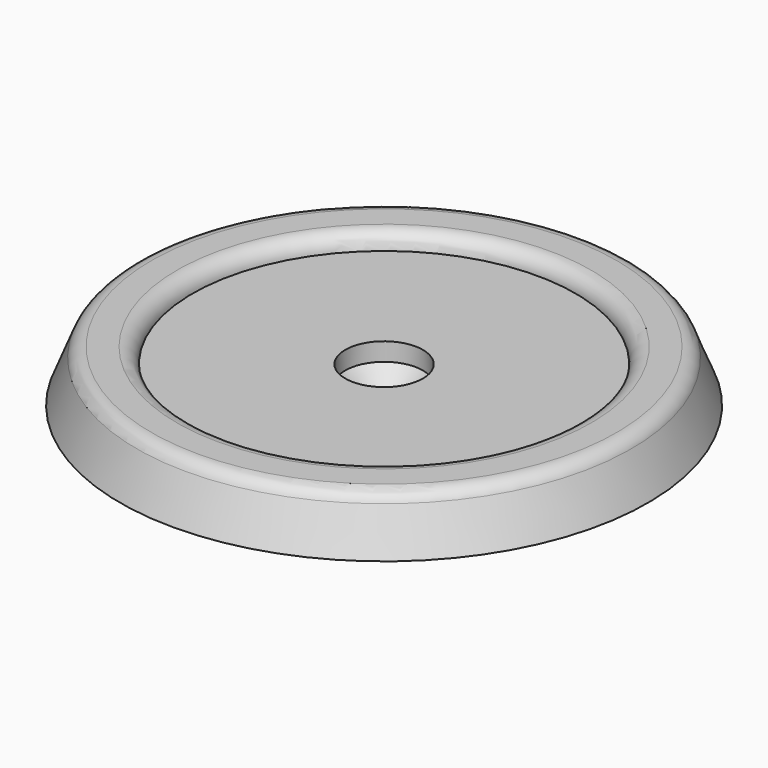
from build123d import *

# Parameters (mm, degrees)
F0_R        = 18.5
F0_R_2      = 2
F1_DEPTH    = 3.5
F2_R        = 3.75
F3_DEPTH    = 0.5
F4_S5_R     = 3.75
F4_T6_DEPTH = 9
F8_R        = 1.49999


# Not quite as in the source:
# - a fillet or chamfer that OpenCascade refuses, or shapes differently, is made with other operations: its cross-section is extruded or revolved along the edge and cut away or added
# - a fillet or chamfer is up to 0.001 mm smaller than in the source, because OpenCascade refuses the exact size


with BuildPart() as f1:
    # F0 (on Top) → F1 (new body)
    with BuildSketch(Plane.XY):
        Circle(F0_R)
        Circle(F0_R_2, mode=Mode.SUBTRACT)
    extrude(amount=F1_DEPTH)

    # F2 (on face) → F3 (cut)
    with BuildSketch(Plane.XY.offset(3.5)):
        Circle(F2_R)
    extrude(amount=-F3_DEPTH, mode=Mode.SUBTRACT)

    # F4: chamfer of 3 on 1 edges, made by hand


with BuildPart() as f4_tool2:
    # F4_s3 → F4_t4 (revolve)
    with BuildSketch(Plane.XZ):
        Polygon((2, 0), (5, 3), (2, 3), align=None)
    revolve(axis=Axis((0, 0, 3), (0, 0, -1)))

    # F4_s5 → F4_t6 (intersect, symmetric)
    with BuildSketch(Plane.XY.offset(1.5)):
        Circle(F4_S5_R)
    extrude(amount=F4_T6_DEPTH, both=True, mode=Mode.INTERSECT)


with BuildPart() as f1_1:
    add(f1.part)

    # F4_t1: cut F4_tool2
    add(f4_tool2.part, mode=Mode.SUBTRACT)

    # F6 (on Right) → F7 (revolve)
    with BuildSketch(Plane.YZ):
        Polygon((-25.5, 0), (-18.5, 0), (-18.5, 3.5), (-18.5, 5), (-23.5, 5), align=None)
    revolve(axis=Axis((0, 0, 7.0907436311), (0, 0, 1)))

    # F8 (radius 1.5 in the source; OpenCascade refuses exactly that, so slightly less here)
    f8_edges = [f1_1.edges().sort_by_distance(p)[0] for p in [
        (0, 23.5, 5),
        (0, 18.5, 5),
    ]]
    fillet(f8_edges, radius=F8_R)


solid = f1_1.part
